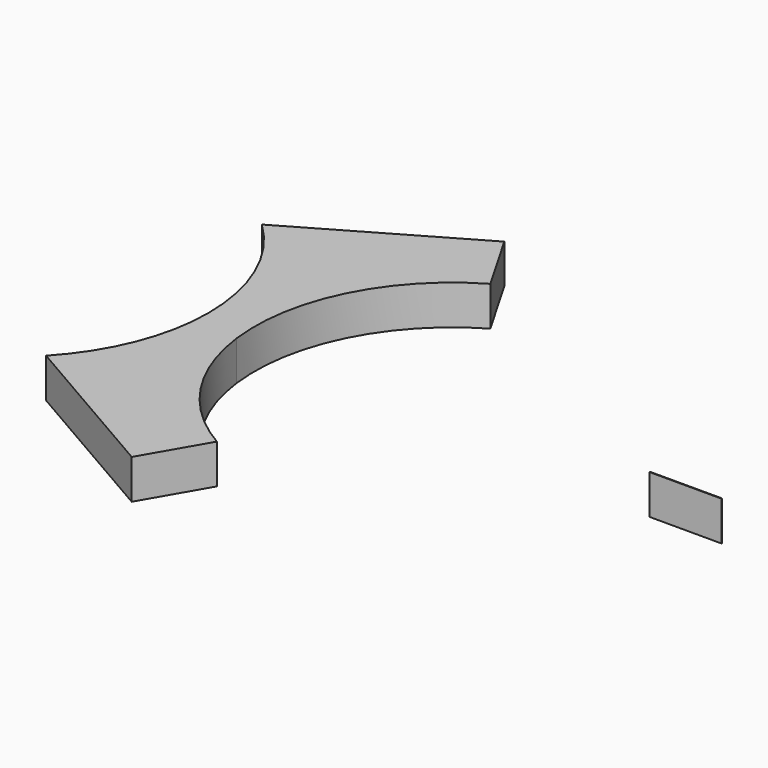
from build123d import *

# Parameters (mm, degrees)
F1_DEPTH = 1.27


# Not quite as in the source:
# - a feature names something its author has since deleted; it is built from what else it names


with BuildPart() as f1:
    # F0 (on Top) → F1 (new body)
    with BuildSketch(Plane.XY):
        with BuildLine():
            ThreePointArc((6.3499692328, 0.0197671951), (6.3499923082, 0.0098836095), (6.35, 0))
            ThreePointArc((6.35, 0), (6.3499999511, -0.0007882849), (6.3499998043, -0.0015765697))
            Line((6.3499998043, -0.0015765697), (8.6649251995, -0.0021513164))
            Line((8.6649251995, -0.0021513164), (8.6649304987, 0.0191924395))
            Line((8.6649304987, 0.0191924395), (6.3499692328, 0.0197671951))
        make_face()
    extrude(amount=F1_DEPTH)


with BuildPart() as f1b:
    # F0 (on Top) → F1, piece 2 (new body)
    with BuildSketch(Plane.XY):
        with BuildLine():
            ThreePointArc((-6.2998185309, -0.7967348855), (-5.6876138678, 2.8237472428), (-3.1736345527, 5.5000494294))
            Line((-3.1736345527, 5.5000494294), (-4.3354020531, 7.5134440315))
            Line((-4.3354020531, 7.5134440315), (-9.6736101808, 4.43319503))
            ThreePointArc((-9.6736101808, 4.43319503), (-8.1076742802, 2.0401198083), (-7.7454316716, -0.7967348855))
            Line((-7.7454316716, -0.7967348855), (-6.2998185309, -0.7967348855))
        make_face()
        with BuildLine():
            Line((-4.3254468713, -7.4875999277), (-3.1763652516, -5.4984728597))
            ThreePointArc((-3.1763652516, -5.4984728597), (-5.28924378, -3.513744475), (-6.2998185309, -0.7967348855))
            Line((-6.2998185309, -0.7967348855), (-7.7454316716, -0.7967348855))
            ThreePointArc((-7.7454316716, -0.7967348855), (-8.2890892892, -2.8029936058), (-9.4496794179, -4.5274263273))
            Line((-9.4496794179, -4.5274263273), (-4.3254468713, -7.4875999277))
        make_face()
    extrude(amount=F1_DEPTH)


solid = Compound([f1.part, f1b.part])
